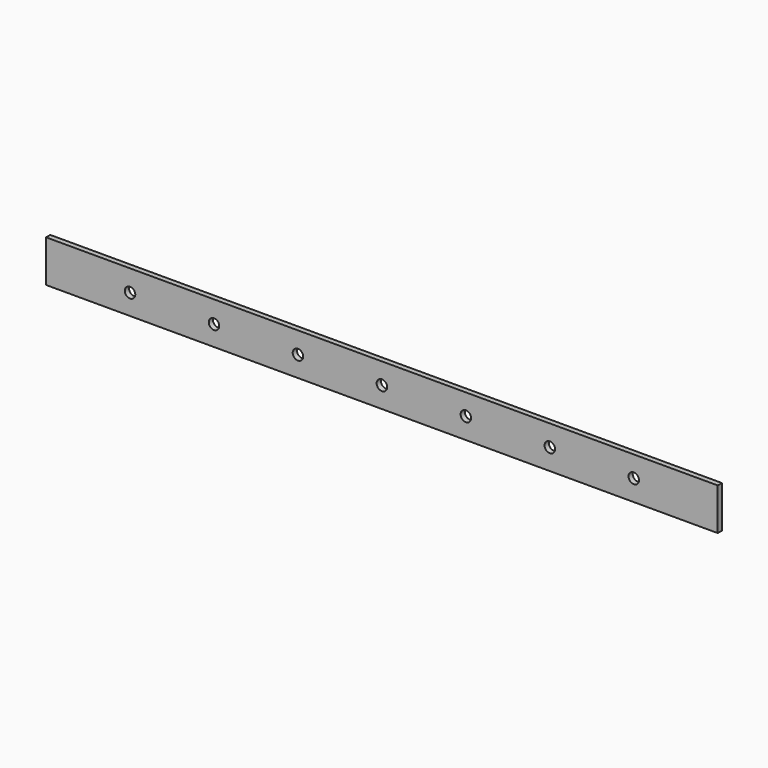
from build123d import *

# Parameters (mm, degrees)
F0_W     = 406.4
F0_H     = 25.4
F0_R     = 3.175
F1_DEPTH = 3.175


# Not quite as in the source:
# - a length typed as a fraction of an inch, garbled in the dataset ("3 / 203.2 mm" for 3/8 in), is restored


with BuildPart() as f1:
    # F0 (on Front) → F1 (new body)
    with BuildSketch(Plane.XZ):
        with Locations((136.8539219917, 1.0073203593)):
            Rectangle(F0_W, F0_H)
        with Locations((-15.5460780083, 0.7554902695)):
            Circle(F0_R, mode=Mode.SUBTRACT)
        with Locations((35.2539219917, 0.5036601797)):
            Circle(F0_R, mode=Mode.SUBTRACT)
        with Locations((86.0539219917, 0.7554902695)):
            Circle(F0_R, mode=Mode.SUBTRACT)
        with Locations((136.8539219917, 1.0073203593)):
            Circle(F0_R, mode=Mode.SUBTRACT)
        with Locations((187.6539219917, 1.0073203593)):
            Circle(F0_R, mode=Mode.SUBTRACT)
        with Locations((238.4539219917, 1.0073203593)):
            Circle(F0_R, mode=Mode.SUBTRACT)
        with Locations((289.2539219917, 1.0073203593)):
            Circle(F0_R, mode=Mode.SUBTRACT)
    extrude(amount=F1_DEPTH)


solid = f1.part
